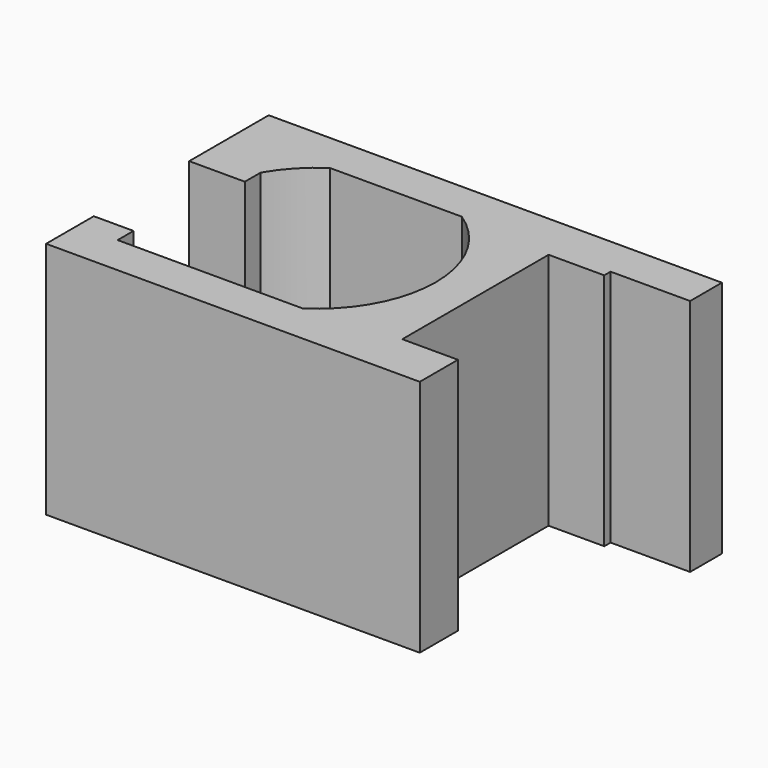
from build123d import *

# Parameters (mm, degrees)
F0_W     = 7
F0_H     = 5
F0_H_2   = 1
F0_W_2   = 10
F0_W_3   = 5
F0_H_3   = 2.5
F1_DEPTH = 30


with BuildPart() as f1:
    # F0 (on Top) → F1 (new body)
    with BuildSketch(Plane.XY):
        with BuildLine():
            Line((20, 12.5), (20, 17.5))
            Line((20, 17.5), (-13, 17.5))
            Line((-13, 17.5), (-13, 12.5))
            Line((-13, 12.5), (-8.2915619759, 12.5))
            ThreePointArc((-8.2915619759, 12.5), (0, 15), (8.2915619759, 12.5))
            Line((8.2915619759, 12.5), (20, 12.5))
        make_face()
        with Locations((23.5, 15)):
            Rectangle(F0_W, F0_H)
        with Locations((-16.5, 15)):
            Rectangle(F0_W, F0_H)
        with Locations((23.5, 12)):
            Rectangle(F0_W, F0_H_2)
        with BuildLine():
            Line((20, 11.5), (20, 12.5))
            Line((20, 12.5), (8.2915619759, 12.5))
            ThreePointArc((8.2915619759, 12.5), (13.2169101843, 7.0931858273), (15, 0))
            ThreePointArc((15, 0), (13.2169101843, -7.0931858273), (8.2915619759, -12.5))
            Line((8.2915619759, -12.5), (20, -12.5))
            Line((20, -12.5), (20, -11.5))
            Line((20, -11.5), (20, 11.5))
        make_face()
        with Locations((32, 15)):
            Rectangle(F0_W_2, F0_H)
        with BuildLine():
            Line((-13, 7.4833147735), (-13, 12.5))
            Line((-13, 12.5), (-20, 12.5))
            Line((-20, 12.5), (-20, 5))
            Line((-20, 5), (-14.1421356237, 5))
            ThreePointArc((-14.1421356237, 5), (-13.627750901, 6.2677272898), (-13, 7.4833147735))
        make_face()
        with BuildLine():
            Line((-8.2915619759, 12.5), (-13, 12.5))
            Line((-13, 12.5), (-13, 7.4833147735))
            ThreePointArc((-13, 7.4833147735), (-10.9372956213, 10.2652600791), (-8.2915619759, 12.5))
        make_face()
        with BuildLine():
            Line((-8.2915619759, 12.5), (8.2915619759, 12.5))
            ThreePointArc((8.2915619759, 12.5), (0, 15), (-8.2915619759, 12.5))
        make_face()
        with BuildLine():
            Line((-13, 5), (-13, 7.4833147735))
            ThreePointArc((-13, 7.4833147735), (-13.627750901, 6.2677272898), (-14.1421356237, 5))
            Line((-14.1421356237, 5), (-13, 5))
        make_face()
        with Locations((23.5, -12)):
            Rectangle(F0_W, F0_H_2)
        with Locations((23.5, -15)):
            Rectangle(F0_W, F0_H)
        with BuildLine():
            Line((20, -17.5), (20, -12.5))
            Line((20, -12.5), (8.2915619759, -12.5))
            ThreePointArc((8.2915619759, -12.5), (4.3301270189, -14.3614066163), (0, -15))
            Line((0, -15), (-15, -15))
            Line((-15, -15), (-15, -17.5))
            Line((-15, -17.5), (20, -17.5))
        make_face()
        with BuildLine():
            ThreePointArc((0, -15), (4.3301270189, -14.3614066163), (8.2915619759, -12.5))
            Line((8.2915619759, -12.5), (-8.2915619759, -12.5))
            ThreePointArc((-8.2915619759, -12.5), (-4.3301270189, -14.3614066163), (0, -15))
        make_face()
        with Locations((-17.5, -11.25)):
            Rectangle(F0_W_3, F0_H_3)
        with BuildLine():
            ThreePointArc((0, -15), (-4.3301270189, -14.3614066163), (-8.2915619759, -12.5))
            Line((-8.2915619759, -12.5), (-15, -12.5))
            Line((-15, -12.5), (-15, -15))
            Line((-15, -15), (0, -15))
        make_face()
        Polygon((-15, -12.5), (-20, -12.5), (-20, -17.5), (-15, -17.5), (-15, -15), align=None)
    extrude(amount=F1_DEPTH)


solid = f1.part
